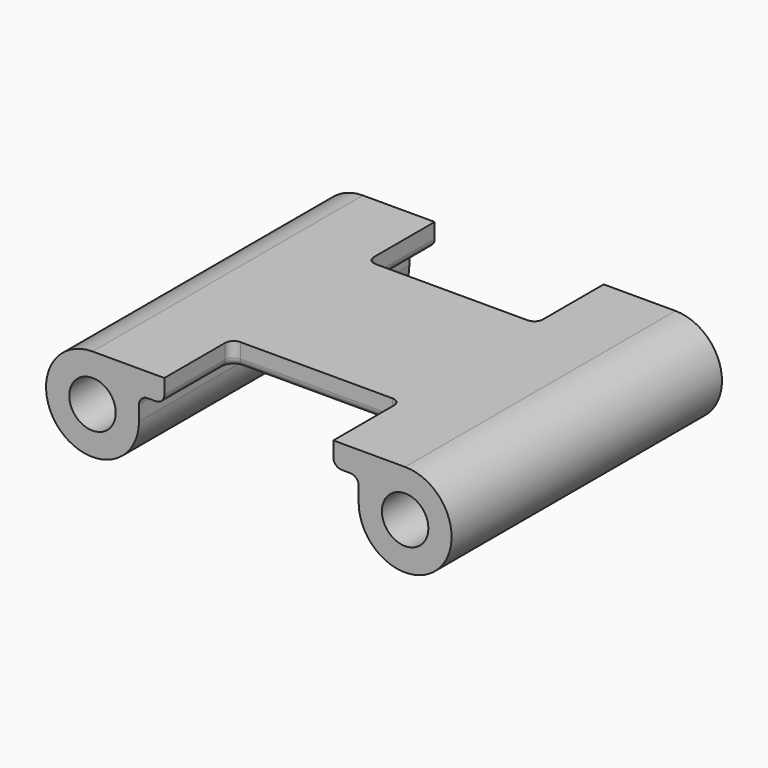
from build123d import *

# Parameters (mm, degrees)
F0_R          = 2.75
F1_DEPTH      = 20
F1_DEPTH_BACK = 20
F2_W          = 20
F2_H          = 10
F3_DEPTH      = 2.75
F4_R          = 1


with BuildPart() as f1:
    # F0 (on Front) → F1 (new body, two sides)
    with BuildSketch(Plane.XZ) as f1_sk:
        with BuildLine():
            Line((37, 5.5), (0, 5.5))
            ThreePointArc((0, 5.5), (-3.8890872965, -3.8890872965), (5.5, 0))
            Line((5.5, 0), (5.5, 1.75))
            ThreePointArc((5.5, 1.75), (5.7928932188, 2.4571067812), (6.5, 2.75))
            Line((6.5, 2.75), (30.5, 2.75))
            ThreePointArc((30.5, 2.75), (31.2071067812, 2.4571067812), (31.5, 1.75))
            Line((31.5, 1.75), (31.5, 0))
            ThreePointArc((31.5, 0), (40.8890872965, -3.8890872965), (37, 5.5))
        make_face()
        Circle(F0_R, mode=Mode.SUBTRACT)
        with Locations((37, 0)):
            Circle(F0_R, mode=Mode.SUBTRACT)
    extrude(amount=F1_DEPTH)
    extrude(f1_sk.sketch, amount=-F1_DEPTH_BACK)

    # F2 (on face) → F3 (cut, through all)
    with BuildSketch(Plane(origin=(0, 0, 2.75), x_dir=(1, 0, 0), z_dir=(0, 0, -1))):
        with Locations((18.5, -15)):
            Rectangle(F2_W, F2_H)
        with Locations((18.5, 15)):
            Rectangle(F2_W, F2_H)
    extrude(amount=-F3_DEPTH, mode=Mode.SUBTRACT)

    # F4
    f4_edges = [f1.edges().sort_by_distance(p)[0] for p in [
        (8.5, -15, 2.75),
        (8.5, 15, 2.75),
        (28.5, 15, 2.75),
        (28.5, -15, 2.75),
        (8.5, -10, 4.125),
        (28.5, -10, 4.125),
        (28.5, 10, 4.125),
        (8.5, 10, 4.125),
        (18.5, 10, 2.75),
        (18.5, -10, 2.75),
    ]]
    fillet(f4_edges, radius=F4_R)


solid = f1.part
